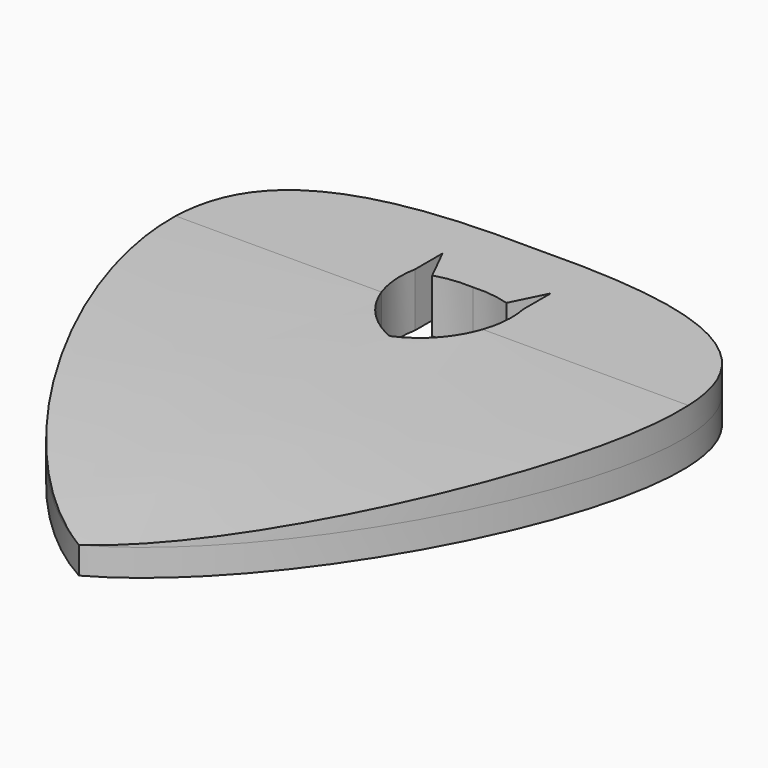
from build123d import *

# Parameters (mm, degrees)
F1_DEPTH = 1.5
F4_DEPTH = 35
F6_DEPTH = 25


with BuildPart() as f1:
    # F0 (on Top) → F1 (new body, symmetric)
    with BuildSketch(Plane.XY):
        with BuildLine():
            add(Edge.make_bspline(
                [(0, 16), (6.1912308447, 16.1269828677), (21.6322143415, 14.6137327369), (8.0521190539, -11.5674184635), (0, -16)],
                knots=[0, 0, 0, 0, 0.4136694367, 1, 1, 1, 1], degree=3))
            add(Edge.make_bspline(
                [(0, 16), (-6.1912308447, 16.1269828677), (-21.6322143415, 14.6137327369), (-8.0521190539, -11.5674184635), (0, -16)],
                knots=[0, 0, 0, 0, 0.4136694367, 1, 1, 1, 1], degree=3))
        make_face()
    extrude(amount=F1_DEPTH, both=True)

    # F3 (on offset) → F4 (cut)
    with BuildSketch(Plane.YZ.offset(15)):
        with BuildLine():
            add(Edge.make_bspline(
                [(-16, 0), (-7.6402679005, 1.0387831861), (0.5034198032, 1.4199266316), (8.633417238, 1.5)],
                knots=[0, 0, 0, 0, 24.6053512698, 24.6053512698, 24.6053512698, 24.6053512698], degree=3))
            Line((8.633417238, 1.5), (-16, 1.5))
            Line((-16, 1.5), (-16, 0))
        make_face()
    extrude(amount=-F4_DEPTH, mode=Mode.SUBTRACT)

    # F5 (on face) → F6 (cut)
    with BuildSketch(Plane.XY.offset(1.5)):
        with BuildLine():
            ThreePointArc((2.0718916785, 11.2373186275), (1.0466922086, 11.4498374057), (0, 11.4750089124))
            ThreePointArc((0, 11.4750089124), (-1.0466922086, 11.4498374057), (-2.0718916785, 11.2373186275))
            Line((-2.0718916785, 11.2373186275), (-3.0199242756, 13.1428707391))
            Line((-3.0199242756, 13.1428707391), (-3.0199242756, 11.2373186275))
            ThreePointArc((-3.0199242756, 11.2373186275), (-3.0933443524, 9.9221413952), (-2.8208159928, 8.633417238))
            Line((-2.8208159928, 8.633417238), (2.8208159928, 8.633417238))
            ThreePointArc((2.8208159928, 8.633417238), (3.0933443524, 9.9221413952), (3.0199242756, 11.2373186275))
            Line((3.0199242756, 11.2373186275), (3.0199242756, 13.1428707391))
            Line((3.0199242756, 13.1428707391), (2.0718916785, 11.2373186275))
        make_face()
        with BuildLine():
            Line((2.8208159928, 8.633417238), (-2.8208159928, 8.633417238))
            ThreePointArc((-2.8208159928, 8.633417238), (-1.7265393737, 6.8526567573), (0, 5.6746877424))
            ThreePointArc((0, 5.6746877424), (1.7265393737, 6.8526567573), (2.8208159928, 8.633417238))
        make_face()
    extrude(amount=-F6_DEPTH, mode=Mode.SUBTRACT)


solid = f1.part
